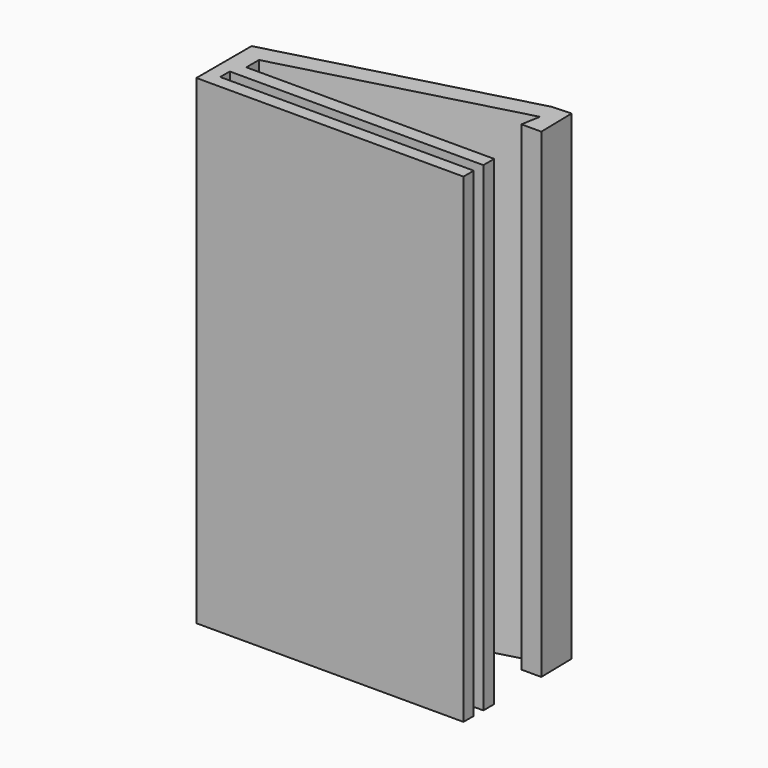
from build123d import *

# Parameters (mm, degrees)
F0_W          = 55.6310900272
F0_H          = 100
F1_DEPTH      = 8
F2_W          = 2.5
F2_H          = 158.0840436167
F3_DEPTH      = 27.8165450136
F3_DEPTH_BACK = 25
F5_DEPTH      = 50


# Not quite as in the source:
# - a feature names something its author has since deleted; it is built from what else it names


with BuildPart() as f1:
    # F0 (on Front) → F1 (new body)
    with BuildSketch(Plane.XZ):
        Rectangle(F0_W, F0_H)
    extrude(amount=-F1_DEPTH)

    # F2 (on Right) → F3 (cut, two sides)
    with BuildSketch(Plane.YZ) as f3_sk:
        with Locations((3.9288233686, 7.7119854566)):
            Rectangle(F2_W, F2_H)
    extrude(amount=F3_DEPTH, mode=Mode.SUBTRACT)
    extrude(f3_sk.sketch, amount=-F3_DEPTH_BACK, mode=Mode.SUBTRACT)

    # F4 (on Top) → F5 (join, symmetric)
    with BuildSketch(Plane.XY):
        Polygon((23.6732276815, 28.1708468052), (-27.8155450136, 14.3744717422), (-27.8155450136, 8), (-23.8155450136, 8), (-23.8155450136, 11.3051637903), (24.3706528022, 24.2166165814), (23.6732276815, 20.2701286405), (27.8155450136, 20.2701286405), (27.6694063807, 28.3456489901), align=None)
    extrude(amount=F5_DEPTH, both=True)


solid = f1.part
